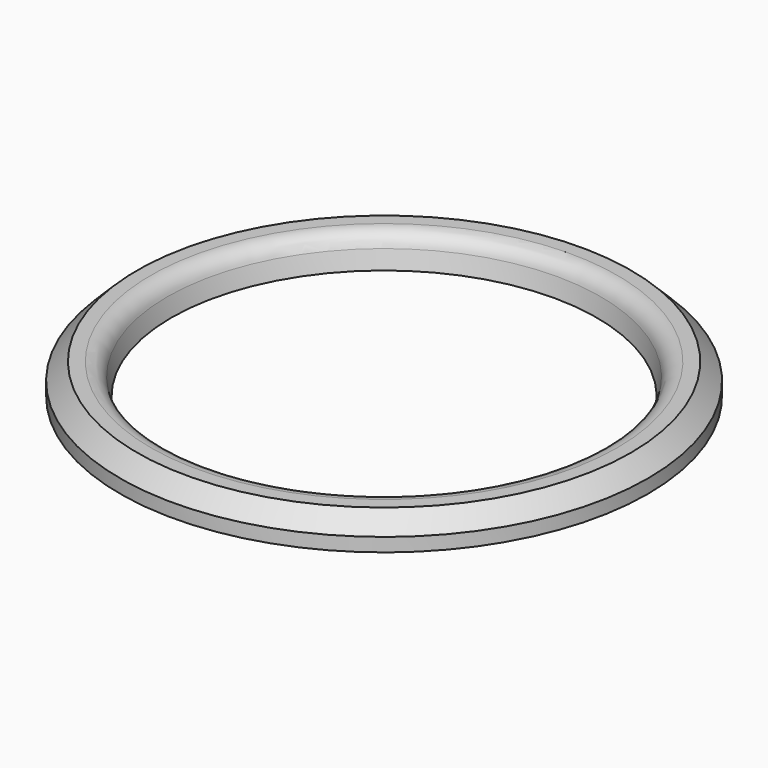
from build123d import *

# Parameters (mm, degrees)
F0_R     = 77.5
F0_R_2   = 62.5
F1_DEPTH = 9
F2_SIZE  = 5
F3_SIZE2 = 1.99999
F3_SIZE  = 8.99999
F4_R     = 5
F5_R     = 5
F6_DEPTH = 5
F7_R     = 2


# Not quite as in the source:
# - a fillet or chamfer is up to 0.001 mm smaller than in the source, because OpenCascade refuses the exact size


with BuildPart() as f1:
    # F0 (on Top) → F1 (new body)
    with BuildSketch(Plane.XY):
        Circle(F0_R)
        Circle(F0_R_2, mode=Mode.SUBTRACT)
    extrude(amount=F1_DEPTH)

    # F2
    f2_edges = [f1.edges().sort_by_distance(p)[0] for p in [
        (-77.5, 0, 9),
    ]]
    chamfer(f2_edges, length=F2_SIZE)

    # F3 (size 9 and 2 in the source; OpenCascade refuses exactly that, so slightly less here)
    f3_edges = [f1.edges().sort_by_distance(p)[0] for p in [
        (-62.5, 0, 9),
    ]]
    f3_side = f1.faces().sort_by_distance((-62.5, 0, 4.5))[0]
    chamfer(f3_edges, length=F3_SIZE, length2=F3_SIZE2, reference=f3_side)

    # F4
    f4_edges = [f1.edges().sort_by_distance(p)[0] for p in [
        (-64.49999, 0, 9),
    ]]
    fillet(f4_edges, radius=F4_R)

    # F5 (on face) → F6 (cut)
    with BuildSketch(Plane(origin=(0, 0, 0), x_dir=(1, 0, 0), z_dir=(0, 0, -1))):
        with Locations((0, 69)):
            Circle(F5_R)
        with Locations((-69, 0)):
            Circle(F5_R)
        with Locations((0, -69)):
            Circle(F5_R)
        with Locations((69, 0)):
            Circle(F5_R)
    extrude(amount=-F6_DEPTH, mode=Mode.SUBTRACT)

    # F7
    f7_edges = [f1.edges().sort_by_distance(p)[0] for p in [
        (-5, -69, 5),
        (-74, 0, 5),
        (64, 0, 5),
        (-5, 69, 5),
    ]]
    fillet(f7_edges, radius=F7_R)


solid = f1.part
